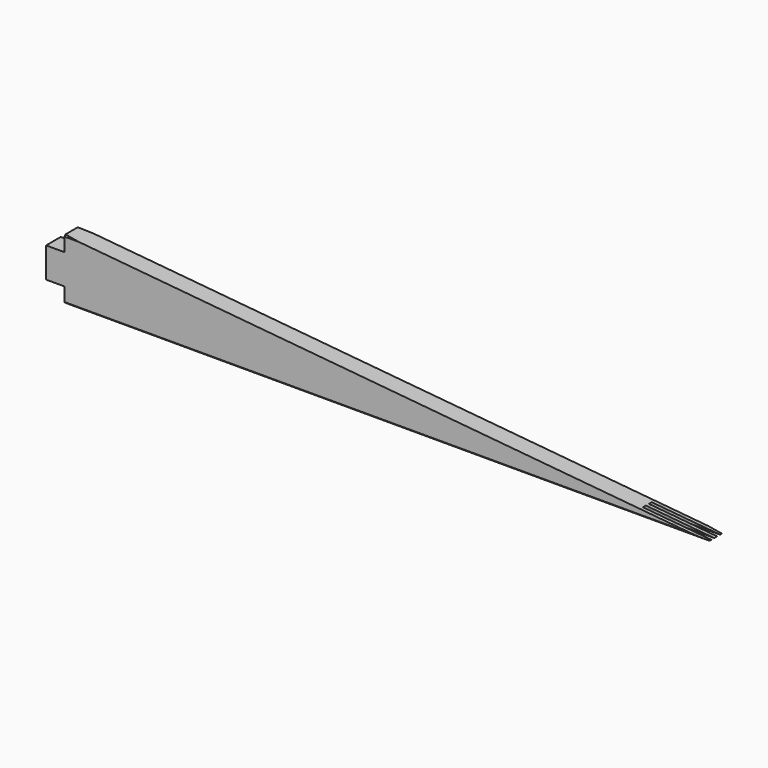
from build123d import *

# Parameters (mm, degrees)
F1_W     = 40
F1_H     = 33
F3_DEPTH = 1275
F2_W     = 80
F2_H     = 100
F4_DEPTH = 25
F6_DEPTH = 50


with BuildPart() as f3:
    # F1 (on Right) → F3 (new body, symmetric)
    with BuildSketch(Plane.YZ):
        Polygon((20, 33), (20, 63), (17, 66), (12, 66), (12, 80), (4, 80), (4, 66), (-4, 66), (-4, 80), (-12, 80), (-12, 66), (-17, 66), (-20, 63), (-20, 33), align=None)
        with Locations((0, 16.5)):
            Rectangle(F1_W, F1_H)
        with Locations((0, -16.5)):
            Rectangle(F1_W, F1_H)
        Polygon((20, -63), (20, -33), (-20, -33), (-20, -63), (-17, -66), (-12, -66), (-12, -52), (-4, -52), (-4, -66), (4, -66), (4, -52), (12, -52), (12, -66), (17, -66), align=None)
    extrude(amount=F3_DEPTH, both=True)

    # F2 (on Front) → F4 (cut, symmetric)
    with BuildSketch(Plane.XZ):
        with Locations((-1275, 83)):
            Rectangle(F2_W, F2_H)
        with Locations((-1275, -83)):
            Rectangle(F2_W, F2_H)
        with Locations((1275, 83)):
            Rectangle(F2_W, F2_H)
        with Locations((1275, -83)):
            Rectangle(F2_W, F2_H)
    extrude(amount=F4_DEPTH, both=True, mode=Mode.SUBTRACT)

    # F5 (on face) → F6 (cut, symmetric)
    with BuildSketch(Plane.XZ.offset(20)):
        Polygon((1525, 88.4753859), (-1475, 88.4753859), (-1202.9649549421, 63), (1235, 63), (1235, 33), (1275, 33), (1275, -33), (1235, -33), (1235, -63), (142.5069374912, -63), (1525, -192.4669378497), align=None)
        Polygon((1235, 63), (-1202.9649549421, 63), (142.5069374912, -63), (1235, -63), (1235, -33), (1275, -33), (1275, 33), (1235, 33), align=None)
    extrude(amount=F6_DEPTH, both=True, mode=Mode.SUBTRACT)


solid = f3.part
